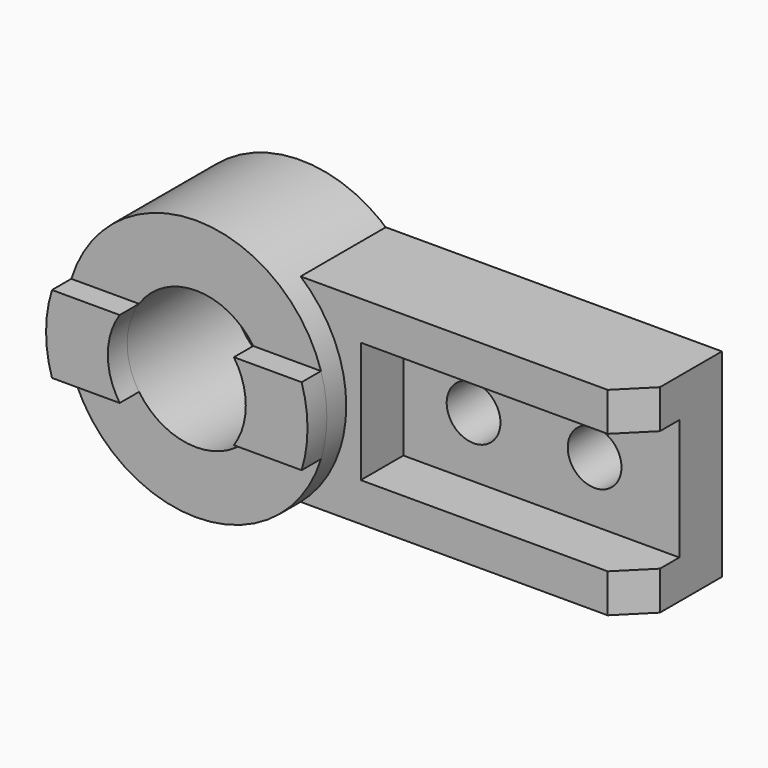
from build123d import *
from build123d import SkipClean  # not in build123d's __all__

# Parameters (mm, degrees)
F0_R      = 54
F0_R_2    = 28.5
F1_DEPTH  = 54
F3_DEPTH  = 10
F5_DEPTH  = 44
F6_W      = 114
F6_H      = 50
F7_DEPTH  = 22
F8_SIZE   = 12
F9_R      = 11.1
F10_DEPTH = 22


with BuildPart() as f1:
    # F0 (on Front) → F1 (new body)
    with BuildSketch(Plane.XZ):
        Circle(F0_R)
        Circle(F0_R_2, mode=Mode.SUBTRACT)
    extrude(amount=-F1_DEPTH)

    # F2 (on Front) → F3 (join)
    with BuildSketch(Plane.XZ):
        with BuildLine():
            ThreePointArc((-23.5849528301, -16), (-28.5, 0), (-23.5849528301, 16))
            Line((-23.5849528301, 16), (-51.5751878329, 16))
            ThreePointArc((-51.5751878329, 16), (-54, 0), (-51.5751878329, -16))
            Line((-51.5751878329, -16), (-23.5849528301, -16))
        make_face()
        with BuildLine():
            Line((51.5751878329, 16), (23.5849528301, 16))
            ThreePointArc((23.5849528301, 16), (28.5, 0), (23.5849528301, -16))
            Line((23.5849528301, -16), (51.5751878329, -16))
            ThreePointArc((51.5751878329, -16), (54, 0), (51.5751878329, 16))
        make_face()
    with SkipClean():  # cleaning this boolean's faces spoils the solid; the shape is the same uncleaned
        extrude(amount=F3_DEPTH)


with BuildPart() as f5:
    # F4 (on face) → F5 (new body)
    with BuildSketch(Plane(origin=(0, 54, 0), x_dir=(-1, 0, 0), z_dir=(0, 1, 0))):
        with BuildLine():
            Line((-174, 41), (-174, 0))
            Line((-174, 0), (-174, -41))
            Line((-174, -41), (-35.1425667816, -41))
            ThreePointArc((-35.1425667816, -41), (-49.0596504584, -22.5643678594), (-54, 0))
            ThreePointArc((-54, 0), (-49.0596504584, 22.5643678594), (-35.1425667816, 41))
            Line((-35.1425667816, 41), (-174, 41))
        make_face()
    extrude(amount=-F5_DEPTH)

    # F6 (on face) → F7 (cut)
    with BuildSketch(Plane.XZ.offset(-10)):
        with Locations((117, 0)):
            Rectangle(F6_W, F6_H)
    extrude(amount=-F7_DEPTH, mode=Mode.SUBTRACT)

    # F8
    f8_edges = [f5.edges().sort_by_distance(p)[0] for p in [
        (174, 10, 33),
        (174, 10, -33),
    ]]
    chamfer(f8_edges, length=F8_SIZE)

    # F9 (on face) → F10 (cut, through all)
    with BuildSketch(Plane.XZ.offset(-32)):
        with Locations((139, 0)):
            Circle(F9_R)
        with Locations((89, 0)):
            Circle(F9_R)
    extrude(amount=-F10_DEPTH, mode=Mode.SUBTRACT)


solid = Compound([f1.part, f5.part])
